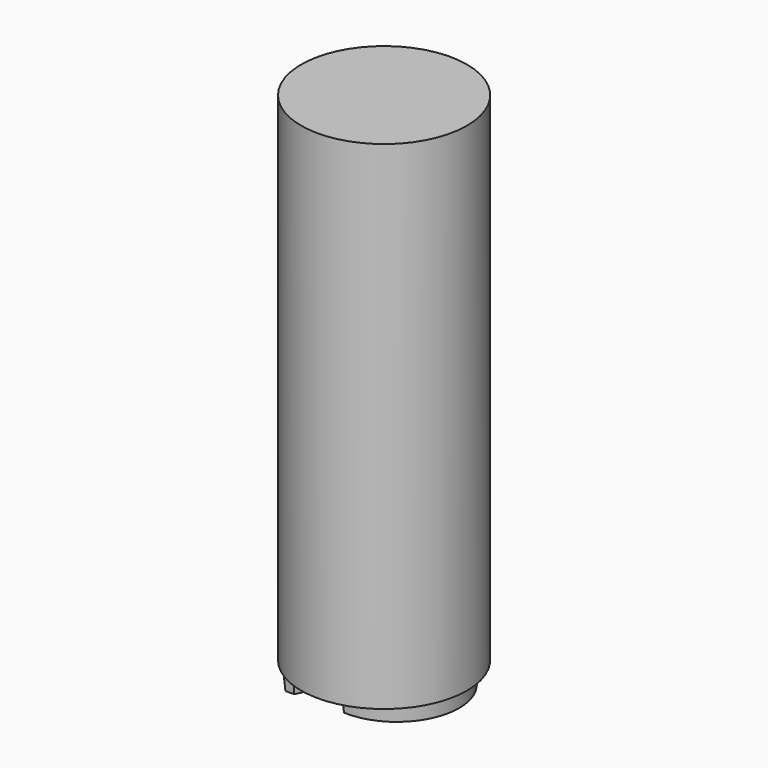
from build123d import *

# Parameters (mm, degrees)
F1_DEPTH = 1.5
F1_TAPER = 3
F0_R     = 5
F2_DEPTH = 30


with BuildPart() as f1:
    # F0 (on Top) → F1 (new body)
    with BuildSketch(Plane.XY):
        with BuildLine():
            ThreePointArc((0, -3.2), (4.103420501, 0.6354360376), (0, 4.4708720751))
            Line((0, 4.4708720751), (-2.0848018873, 0))
            Line((-2.0848018873, 0), (-3.9100516587, 0))
            ThreePointArc((-3.9100516587, 0), (-4.1221836931, -0.0878679656), (-4.2100516587, -0.3))
            Line((-4.2100516587, -0.3), (-4.2100516587, -0.4))
            ThreePointArc((-4.2100516587, -0.4), (-4.1221836931, -0.6121320344), (-3.9100516587, -0.7))
            Line((-3.9100516587, -0.7), (-2.411217248, -0.7))
            Line((-2.411217248, -0.7), (-3.5769863934, -3.2))
            Line((-3.5769863934, -3.2), (-2.8769863934, -3.2))
            Line((-2.8769863934, -3.2), (-1.711217248, -0.7))
            Line((-1.711217248, -0.7), (0, -0.7))
            Line((0, -0.7), (0, -3.2))
        make_face()
        Polygon((0, 0), (-1.3848018873, 0), (0, 2.9697172308), align=None, mode=Mode.SUBTRACT)
        with BuildLine():
            Line((0.7, -2.4777031195), (0.7, 3.7485751946))
            ThreePointArc((0.7, 3.7485751946), (3.403420501, 0.6354360376), (0.7, -2.4777031195))
        make_face(mode=Mode.SUBTRACT)
    extrude(amount=-F1_DEPTH, taper=F1_TAPER)


with BuildPart() as f2:
    # F0 (on Top) → F2 (new body)
    with BuildSketch(Plane.XY):
        Circle(F0_R)
        with BuildLine():
            Line((-2.0848018873, 0), (0, 4.4708720751))
            ThreePointArc((0, 4.4708720751), (4.103420501, 0.6354360376), (0, -3.2))
            Line((0, -3.2), (0, -0.7))
            Line((0, -0.7), (-1.711217248, -0.7))
            Line((-1.711217248, -0.7), (-2.8769863934, -3.2))
            Line((-2.8769863934, -3.2), (-3.5769863934, -3.2))
            Line((-3.5769863934, -3.2), (-2.411217248, -0.7))
            Line((-2.411217248, -0.7), (-3.9100516587, -0.7))
            ThreePointArc((-3.9100516587, -0.7), (-4.1221836931, -0.6121320344), (-4.2100516587, -0.4))
            Line((-4.2100516587, -0.4), (-4.2100516587, -0.3))
            ThreePointArc((-4.2100516587, -0.3), (-4.1221836931, -0.0878679656), (-3.9100516587, 0))
            Line((-3.9100516587, 0), (-2.0848018873, 0))
        make_face(mode=Mode.SUBTRACT)
        with BuildLine():
            ThreePointArc((0, -3.2), (4.103420501, 0.6354360376), (0, 4.4708720751))
            Line((0, 4.4708720751), (-2.0848018873, 0))
            Line((-2.0848018873, 0), (-3.9100516587, 0))
            ThreePointArc((-3.9100516587, 0), (-4.1221836931, -0.0878679656), (-4.2100516587, -0.3))
            Line((-4.2100516587, -0.3), (-4.2100516587, -0.4))
            ThreePointArc((-4.2100516587, -0.4), (-4.1221836931, -0.6121320344), (-3.9100516587, -0.7))
            Line((-3.9100516587, -0.7), (-2.411217248, -0.7))
            Line((-2.411217248, -0.7), (-3.5769863934, -3.2))
            Line((-3.5769863934, -3.2), (-2.8769863934, -3.2))
            Line((-2.8769863934, -3.2), (-1.711217248, -0.7))
            Line((-1.711217248, -0.7), (0, -0.7))
            Line((0, -0.7), (0, -3.2))
        make_face()
        Polygon((0, 0), (-1.3848018873, 0), (0, 2.9697172308), align=None, mode=Mode.SUBTRACT)
        with BuildLine():
            Line((0.7, -2.4777031195), (0.7, 3.7485751946))
            ThreePointArc((0.7, 3.7485751946), (3.403420501, 0.6354360376), (0.7, -2.4777031195))
        make_face(mode=Mode.SUBTRACT)
        Polygon((0, 2.9697172308), (-1.3848018873, 0), (0, 0), align=None)
        with BuildLine():
            ThreePointArc((0.7, -2.4777031195), (3.403420501, 0.6354360376), (0.7, 3.7485751946))
            Line((0.7, 3.7485751946), (0.7, -2.4777031195))
        make_face()
    extrude(amount=F2_DEPTH)


solid = Compound([f1.part, f2.part])
